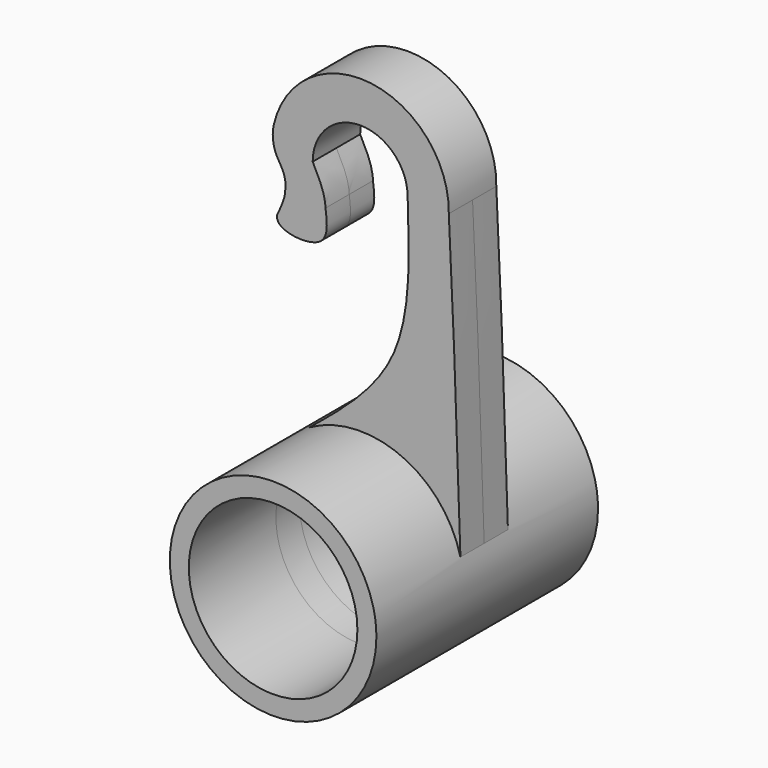
from build123d import *

# Parameters (mm, degrees)
F0_R     = 13.5255
F1_DEPTH = 22.225
F2_DEPTH = 4.7625


with BuildPart() as f1:
    # F0 (on Front) → F1 (new body, symmetric)
    with BuildSketch(Plane.XZ):
        with BuildLine():
            ThreePointArc((16.0855769131, 3.991881464), (6.5567714231, 15.2213550893), (-8.1495274532, 14.4314276681))
            ThreePointArc((-8.1495274532, 14.4314276681), (-8.3550795629, -14.3134044779), (16.5735, 0))
            ThreePointArc((16.5735, 0), (16.4510670052, 2.0107950269), (16.0855769131, 3.991881464))
        make_face()
        Circle(F0_R, mode=Mode.SUBTRACT)
    extrude(amount=F1_DEPTH, both=True)

    # F0 (on Front) → F2 (join, symmetric)
    with BuildSketch(Plane.XZ):
        with BuildLine():
            ThreePointArc((16.0855769131, 3.991881464), (6.5567714231, 15.2213550893), (-8.1495274532, 14.4314276681))
            ThreePointArc((-8.1495274532, 14.4314276681), (-8.3550795629, -14.3134044779), (16.5735, 0))
            ThreePointArc((16.5735, 0), (16.4510670052, 2.0107950269), (16.0855769131, 3.991881464))
        make_face()
        Circle(F0_R, mode=Mode.SUBTRACT)
        with BuildLine():
            add(Edge.make_bspline(
                [(7.6196315943, 52.0585709196), (7.9073561804, 43.8512833929), (8.4668828165, 27.9749976478), (-2.735262235, 18.8402392219), (-8.1495274532, 14.4314276681)],
                knots=[0, 0, 0, 0, 0.5168803488, 1, 1, 1, 1], degree=3))
            ThreePointArc((-8.1495274532, 14.4314276681), (6.5567714231, 15.2213550893), (16.0855769131, 3.991881464))
            add(Edge.make_bspline(
                [(14.2219077444, 51.8895407599), (14.4256822763, 47.7682077132), (14.9759634895, 37.2014626867), (15.653478831, 16.5725180559), (16.0855769131, 3.991881464)],
                knots=[0, 0, 0, 0, 0.3900119934, 1, 1, 1, 1], degree=3))
            ThreePointArc((14.2219077444, 51.8895407599), (1.6964946006, 66.2559672798), (-13.8750644733, 55.2647556367))
            ThreePointArc((-13.8750644733, 55.2647556367), (-13.937377269, 52.7814096229), (-13.0421995878, 50.4641812725))
            add(Edge.make_bspline(
                [(-13.0421995878, 50.4641812725), (-12.3253096001, 49.3346329312), (-11.8330637514, 48.1700341933), (-12.0167843997, 46.8999668956)],
                knots=[0.0832842621, 0.0832842621, 0.0832842621, 0.0832842621, 0.2506068983, 0.2506068983, 0.2506068983, 0.2506068983], degree=3))
            add(Edge.make_bspline(
                [(-12.0167843975, 46.8999668404), (-11.9685081536, 45.6929371066), (-12.6474764459, 44.2057904092), (-13.352232419, 42.7222704399)],
                knots=[0.6168006178, 0.6168006178, 0.6168006178, 0.6168006178, 1, 1, 1, 1], degree=3))
            add(Edge.make_bspline(
                [(-13.352232419, 42.7222704399), (-13.3723404879, 42.3903517549), (-13.0294229695, 40.5231715226), (-8.3379146473, 40.1111053623), (-6.5978615691, 41.1531167984)],
                knots=[0.4383260576, 0.4383260576, 0.4383260576, 0.4383260576, 0.4904587097, 0.7585657185, 0.7585657185, 0.7585657185, 0.7585657185], degree=3))
            add(Edge.make_bspline(
                [(-5.5660903454, 46.2477467954), (-5.5050556705, 44.6482001002), (-5.9652585792, 42.9216600644), (-6.5978615691, 41.1531167984)],
                knots=[0.4687776215, 0.4687776215, 0.4687776215, 0.4687776215, 0.8242974336, 0.8242974336, 0.8242974336, 0.8242974336], degree=3))
            add(Edge.make_bspline(
                [(-7.62, 52.1335), (-6.6332844065, 50.2451802325), (-5.6465688131, 48.356860465), (-5.5660903454, 46.2477467954)],
                knots=[0, 0, 0, 0, 0.4687776215, 0.4687776215, 0.4687776215, 0.4687776215], degree=3))
            ThreePointArc((-7.62, 52.1335), (0.037464993, 59.753407898), (7.6196315943, 52.0585709196))
        make_face()
        with BuildLine():
            add(Edge.make_bspline(
                [(-6.5978615691, 41.1531167984), (-6.5808454576, 41.1633067076), (-5.0331676538, 42.1138674091), (-5.3010837075, 44.1920912662), (-5.5660903454, 46.2477467954)],
                knots=[0.7585657185, 0.7585657185, 0.7585657185, 0.7585657185, 0.7611875574, 1, 1, 1, 1], degree=3))
            add(Edge.make_bspline(
                [(-5.5660903454, 46.2477467954), (-5.5050556705, 44.6482001002), (-5.9652585792, 42.9216600644), (-6.5978615691, 41.1531167984)],
                knots=[0.4687776215, 0.4687776215, 0.4687776215, 0.4687776215, 0.8242974336, 0.8242974336, 0.8242974336, 0.8242974336], degree=3))
        make_face()
    extrude(amount=F2_DEPTH, both=True)


solid = f1.part
